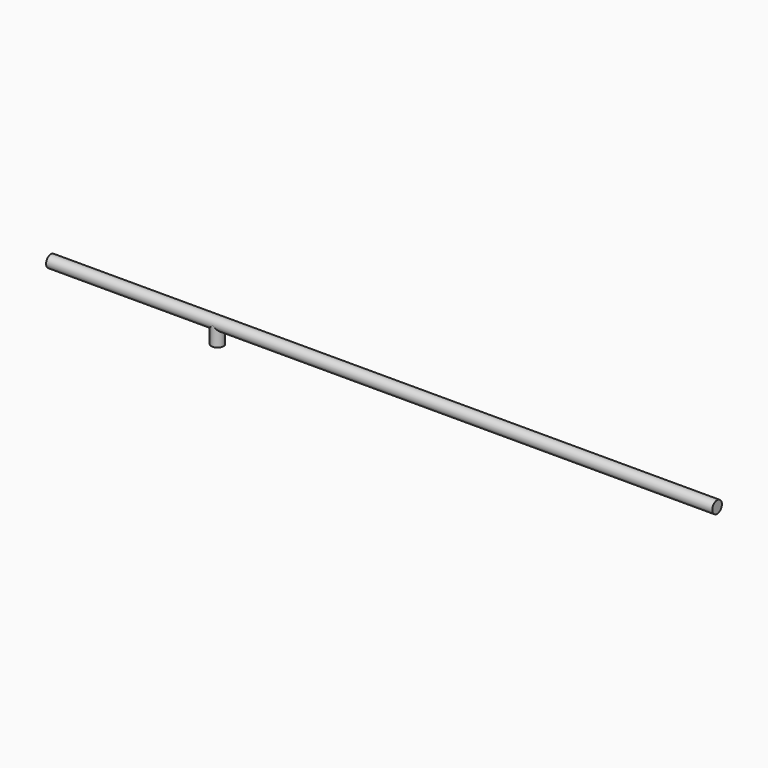
from build123d import *

# Parameters (mm, degrees)
F0_R     = 12.7
F1_DEPTH = 1200
F2_R     = 12.7
F3_DEPTH = 40
F4_DEPTH = 200


with BuildPart() as f1:
    # F0 (on Right) → F1 (new body)
    with BuildSketch(Plane.YZ):
        Circle(F0_R)
    extrude(amount=-F1_DEPTH)

    # F2 (on Top) → F3 (join)
    with BuildSketch(Plane.XY):
        with Locations((-850, 0)):
            Circle(F2_R)
    extrude(amount=-F3_DEPTH)

    # F4 (add): a face of the model
    f4_faces = [f1.faces().sort_by_distance(p)[0] for p in [
        (0, 0, 0),
    ]]
    extrude(f4_faces, amount=F4_DEPTH)


solid = f1.part
